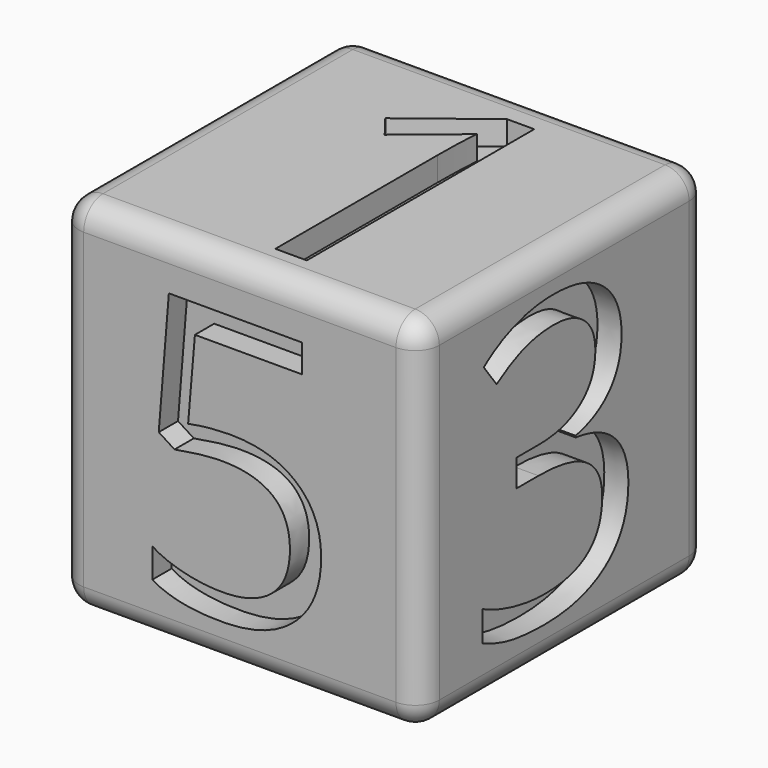
from build123d import *

# Parameters (mm, degrees)
F0_W          = 19
F0_H          = 19
F1_DEPTH      = 19
F2_R          = 1.27
F3_R          = 1.27
F4_R          = 1.27
F5_R          = 1.27
F6_R          = 1.27
F7_TEXT_SIZE  = 20.988537128
F8_DEPTH      = 1.27
F11_TEXT_SIZE = 20.075991698
F12_DEPTH     = 1.27
F10_TEXT_SIZE = 20.5651375129
F14_DEPTH     = 1.27
F13_TEXT_SIZE = 20.6418726723
F15_DEPTH     = 1.27
F16_DEPTH     = 1.27
F17_W         = 16.46
F17_H         = 16.46
F18_DEPTH     = 1.27
F19_TEXT_SIZE = 19.8074470973
F20_DEPTH     = 1.27


# Not quite as in the source:
# - Text() gives the source's letters only with a copy of the font that has no kerning and outlines rounded to 1/6400 em; it was checked with that copy


with BuildPart() as f1:
    # F0 (on Top) → F1 (new body)
    with BuildSketch(Plane.XY):
        with Locations((0.6250813603, -0.8427849505)):
            Rectangle(F0_W, F0_H)
    extrude(amount=F1_DEPTH)

    # F2
    f2_edges = [f1.edges().sort_by_distance(p)[0] for p in [
        (-8.874919, 8.657215, 9.5),
    ]]
    fillet(f2_edges, radius=F2_R)

    # F3
    f3_edges = [f1.edges().sort_by_distance(p)[0] for p in [
        (1.260081, 8.657215, 19),
    ]]
    fillet(f3_edges, radius=F3_R)

    # F4
    f4_edges = [f1.edges().sort_by_distance(p)[0] for p in [
        (10.125081, 8.657215, 8.865),
    ]]
    fillet(f4_edges, radius=F4_R)

    # F5
    f5_edges = [f1.edges().sort_by_distance(p)[0] for p in [
        (0.625081, 8.657215, 0),
    ]]
    fillet(f5_edges, radius=F5_R)

    # F6
    f6_edges = [f1.edges().sort_by_distance(p)[0] for p in [
        (0.625081, -10.342785, 19),
    ]]
    fillet(f6_edges, radius=F6_R)

    # F7 (on face) → F8 (cut)
    with BuildSketch(Plane.XY.offset(19)):
        with Locations((-4.6629402786, -8.4759918973)):
            Text('1', F7_TEXT_SIZE, font='Open Sans', text_align=(TextAlign.LEFT, TextAlign.BOTTOM))
    extrude(amount=-F8_DEPTH, mode=Mode.SUBTRACT)

    # F11 (on face) → F12 (cut)
    with BuildSketch(Plane(origin=(0, 0, 0), x_dir=(1, 0, 0), z_dir=(0, 0, -1))):
        with Locations((-4.9319593236, -6.523238495)):
            Text('6', F11_TEXT_SIZE, font='Open Sans', text_align=(TextAlign.LEFT, TextAlign.BOTTOM))
    extrude(amount=-F12_DEPTH, mode=Mode.SUBTRACT)

    # F10 (on face) → F14 (cut)
    with BuildSketch(Plane.YZ.offset(10.1250813603)):
        with Locations((-7.167806034, 2.1502182353)):
            Text('3', F10_TEXT_SIZE, font='Open Sans', text_align=(TextAlign.LEFT, TextAlign.BOTTOM))
    extrude(amount=-F14_DEPTH, mode=Mode.SUBTRACT)

    # F13 (on face) → F15 (cut)
    with BuildSketch(Plane(origin=(-8.8749186397, 0, 0), x_dir=(0, -1, 0), z_dir=(-1, 0, 0))):
        with Locations((-6.292654667, 2.0922140684)):
            Text('4', F13_TEXT_SIZE, font='Open Sans', text_align=(TextAlign.LEFT, TextAlign.BOTTOM))
        with BuildLine():
            Line((-4.186538596, 7.0011094133), (1.3061347104, 7.0011094133))
            Line((1.3061347104, 7.0011094133), (1.3061347104, 11.9003288803))
            add(Edge.make_bspline(
                [(1.3061347104, 11.9003288803), (1.3061347104, 13.3420346748), (1.4093440738, 15.1546491188)],
                knots=[0, 0, 0, 1, 1, 1], degree=2))
            Line((1.4093440738, 15.1546491188), (1.3287117587, 15.1546491188))
            add(Edge.make_bspline(
                [(1.3287117587, 15.1546491188), (0.8449178679, 14.1870613373), (0.419179244, 13.5516786941)],
                knots=[0, 0, 0, 1, 1, 1], degree=2))
            Line((0.419179244, 13.5516786941), (-4.186538596, 7.0011094133))
        make_face()
    extrude(amount=-F15_DEPTH, mode=Mode.SUBTRACT)

    # F9 (on face) → F16 (cut)
    with BuildSketch(Plane(origin=(0, 8.6572150495, 0), x_dir=(-1, 0, 0), z_dir=(0, 1, 0))):
        with BuildLine():
            Line((-5.3145247418, 3.0717210979), (4.2381687354, 3.0717210979))
            Line((4.2381687354, 3.0717210979), (4.2381687354, 4.6018062003))
            Line((4.2381687354, 4.6018062003), (-3.2372990207, 4.6018062003))
            Line((-3.2372990207, 4.6018062003), (-3.2372990207, 4.6813324531))
            Line((-3.2372990207, 4.6813324531), (-0.0562489117, 7.7923994596))
            add(Edge.make_bspline(
                [(2.8448687876, 11.2120283268), (2.068692561, 9.8600820304), (-0.0562489117, 7.7923994596)],
                knots=[0, 0, 0, 1, 1, 1], degree=2))
            add(Edge.make_bspline(
                [(3.6210450142, 13.9477314205), (3.6210450142, 12.5639746231), (2.8448687876, 11.2120283268)],
                knots=[0, 0, 0, 1, 1, 1], degree=2))
            add(Edge.make_bspline(
                [(2.4583711994, 16.7645512919), (3.6210450142, 15.716395281), (3.6210450142, 13.9477314205)],
                knots=[0, 0, 0, 1, 1, 1], degree=2))
            add(Edge.make_bspline(
                [(0.3281157776, 17.73), (1.6222978927, 17.518275381), (2.4583711994, 16.7645512919)],
                knots=[0.2809046733, 0.2809046733, 0.2809046733, 1, 1, 1], degree=2))
            Line((0.3281157776, 17.73), (-1.788465955, 17.73))
            add(Edge.make_bspline(
                [(-5.1268427854, 16.1426559956), (-3.5662908473, 17.4410549933), (-1.788465955, 17.73)],
                knots=[0, 0, 0, 0.7774605439, 0.7774605439, 0.7774605439], degree=2))
            Line((-5.1268427854, 16.1426559956), (-4.2520540054, 15.0197453072))
            add(Edge.make_bspline(
                [(-2.4483985937, 16.1044833943), (-3.2595663714, 15.8054646841), (-4.2520540054, 15.0197453072)],
                knots=[0, 0, 0, 1, 1, 1], degree=2))
            add(Edge.make_bspline(
                [(-0.7338125849, 16.4035021046), (-1.6372308159, 16.4035021046), (-2.4483985937, 16.1044833943)],
                knots=[0, 0, 0, 1, 1, 1], degree=2))
            add(Edge.make_bspline(
                [(1.2257142822, 15.7227573812), (0.519521158, 16.4035021046), (-0.7338125849, 16.4035021046)],
                knots=[0, 0, 0, 1, 1, 1], degree=2))
            add(Edge.make_bspline(
                [(1.9319074064, 13.8777483181), (1.9319074064, 15.0420126579), (1.2257142822, 15.7227573812)],
                knots=[0, 0, 0, 1, 1, 1], degree=2))
            add(Edge.make_bspline(
                [(1.6535655218, 12.3381200653), (1.9319074064, 13.0538563398), (1.9319074064, 13.8777483181)],
                knots=[0, 0, 0, 1, 1, 1], degree=2))
            add(Edge.make_bspline(
                [(0.8185398682, 10.8668843899), (1.3752236373, 11.6223837908), (1.6535655218, 12.3381200653)],
                knots=[0, 0, 0, 1, 1, 1], degree=2))
            add(Edge.make_bspline(
                [(-1.4877214608, 8.3395400784), (0.2618560992, 10.1113849891), (0.8185398682, 10.8668843899)],
                knots=[0, 0, 0, 1, 1, 1], degree=2))
            Line((-1.4877214608, 8.3395400784), (-5.3145247418, 4.4936504966))
            Line((-5.3145247418, 4.4936504966), (-5.3145247418, 3.0717210979))
        make_face()
    extrude(amount=-F16_DEPTH, mode=Mode.SUBTRACT)

    # F17 (on face) → F18 (join)
    with BuildSketch(Plane.XZ.offset(10.3427849505)):
        with Locations((0.6250813603, 9.5)):
            Rectangle(F17_W, F17_H)
        with BuildLine():
            add(Edge.make_bspline(
                [(-1.8019144784, 10.8307976927), (-0.6479771877, 11.0622280128), (0.4995314829, 11.0622280128)],
                knots=[0, 0, 0, 1, 1, 1], degree=2))
            add(Edge.make_bspline(
                [(0.4995314829, 11.0622280128), (2.8202633042, 11.0622280128), (4.1509876449, 9.9115050322)],
                knots=[0, 0, 0, 1, 1, 1], degree=2))
            add(Edge.make_bspline(
                [(4.1509876449, 9.9115050322), (5.4817119856, 8.7607820516), (5.4817119856, 6.7614812305)],
                knots=[0, 0, 0, 1, 1, 1], degree=2))
            add(Edge.make_bspline(
                [(5.4817119856, 6.7614812305), (5.4817119856, 4.4825354392), (4.0304510198, 3.1855613535)],
                knots=[0, 0, 0, 1, 1, 1], degree=2))
            add(Edge.make_bspline(
                [(4.0304510198, 3.1855613535), (2.579190054, 1.8885872678), (0.0270279126, 1.8885872678)],
                knots=[0, 0, 0, 1, 1, 1], degree=2))
            add(Edge.make_bspline(
                [(0.0270279126, 1.8885872678), (-2.4544194087, 1.8885872678), (-3.7594292694, 2.6825218382)],
                knots=[0, 0, 0, 1, 1, 1], degree=2))
            Line((-3.7594292694, 2.6825218382), (-3.7594292694, 4.2896768391))
            add(Edge.make_bspline(
                [(-3.7594292694, 4.2896768391), (-3.0587096891, 3.8396734389), (-2.0140589385, 3.5825286387)],
                knots=[0, 0, 0, 1, 1, 1], degree=2))
            add(Edge.make_bspline(
                [(-2.0140589385, 3.5825286387), (-0.9694081879, 3.3253838386), (0.0463137727, 3.3253838386)],
                knots=[0, 0, 0, 1, 1, 1], degree=2))
            add(Edge.make_bspline(
                [(0.0463137727, 3.3253838386), (1.8141842736, 3.3253838386), (2.7929416692, 4.159497284)],
                knots=[0, 0, 0, 1, 1, 1], degree=2))
            add(Edge.make_bspline(
                [(2.7929416692, 4.159497284), (3.7716990647, 4.9936107295), (3.7716990647, 6.5718369404)],
                knots=[0, 0, 0, 1, 1, 1], degree=2))
            add(Edge.make_bspline(
                [(3.7716990647, 6.5718369404), (3.7716990647, 9.6447173021), (0.0077420526, 9.6447173021)],
                knots=[0, 0, 0, 1, 1, 1], degree=2))
            add(Edge.make_bspline(
                [(0.0077420526, 9.6447173021), (-0.9469080179, 9.6447173021), (-2.5444200888, 9.3522150919)],
                knots=[0, 0, 0, 1, 1, 1], degree=2))
            Line((-2.5444200888, 9.3522150919), (-3.4090694793, 9.9050764122))
            Line((-3.4090694793, 9.9050764122), (-2.8562081589, 16.777271196))
            Line((-2.8562081589, 16.777271196), (4.4467041651, 16.777271196))
            Line((4.4467041651, 16.777271196), (4.4467041651, 15.2408310151))
            Line((4.4467041651, 15.2408310151), (-1.4290545182, 15.2408310151))
            Line((-1.4290545182, 15.2408310151), (-1.8019144784, 10.8307976927))
        make_face(mode=Mode.SUBTRACT)
    extrude(amount=-F18_DEPTH)

    # F19 (on face) → F20 (cut)
    with BuildSketch(Plane.XZ.offset(10.3427849505)):
        with Locations((-5.2739297971, 2.2135388572)):
            Text('5', F19_TEXT_SIZE, font='Open Sans', text_align=(TextAlign.LEFT, TextAlign.BOTTOM))
    extrude(amount=-F20_DEPTH, mode=Mode.SUBTRACT)


solid = f1.part
